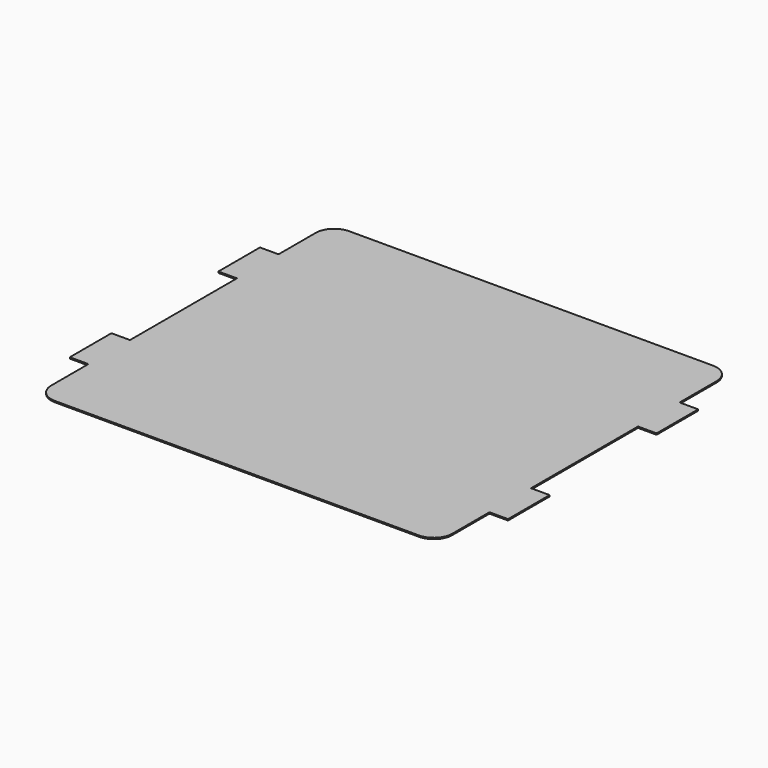
from build123d import *

# Parameters (mm, degrees)
F0_W     = 5
F0_H     = 14
F0_W_2   = 108
F1_DEPTH = 0.35


with BuildPart() as f1:
    # F0 (on Top) → F1 (new body)
    with BuildSketch(Plane.XY):
        with BuildLine():
            ThreePointArc((54, 44.5), (52.5355339059, 48.0355339059), (49, 49.5))
            Line((49, 49.5), (-49, 49.5))
            ThreePointArc((-49, 49.5), (-52.5355339059, 48.0355339059), (-54, 44.5))
            Line((-54, 44.5), (-54, 32))
            Line((-54, 32), (54, 32))
            Line((54, 32), (54, 44.5))
        make_face()
        with Locations((56.5, 25)):
            Rectangle(F0_W, F0_H)
        Polygon((54, 18), (54, 32), (-54, 32), (-54, 18), (0, 18), align=None)
        with Locations((-56.5, 25)):
            Rectangle(F0_W, F0_H)
        Polygon((54, -18), (54, 18), (0, 18), (-54, 18), (-54, -18), align=None)
        with Locations((56.5, -25)):
            Rectangle(F0_W, F0_H)
        with Locations((0, -25)):
            Rectangle(F0_W_2, F0_H)
        with Locations((-56.5, -25)):
            Rectangle(F0_W, F0_H)
        with BuildLine():
            Line((54, -44.5), (54, -32))
            Line((54, -32), (-54, -32))
            Line((-54, -32), (-54, -44.5))
            ThreePointArc((-54, -44.5), (-52.5355339059, -48.0355339059), (-49, -49.5))
            Line((-49, -49.5), (49, -49.5))
            ThreePointArc((49, -49.5), (52.5355339059, -48.0355339059), (54, -44.5))
        make_face()
    extrude(amount=F1_DEPTH)


solid = f1.part
